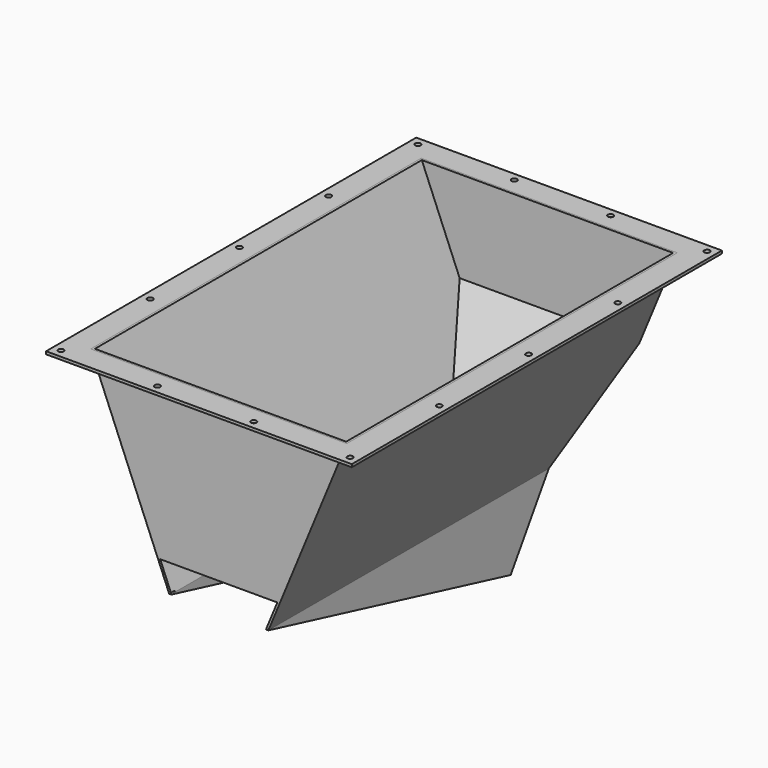
from build123d import *

# Parameters (mm, degrees)
F1_DEPTH  = 1500
F2_W      = 1110
F2_H      = 1680
F2_W_2    = 930
F2_H_2    = 1500
F3_DEPTH  = 10
F4_R      = 10
F5_DEPTH  = 10
F7_DEPTH  = 1110.001
F8_T      = -8
F10_DEPTH = 8
F11_W     = 344
F11_H     = 1124.6517558367
F12_DEPTH = 8


with BuildPart() as f1:
    # F0 (on Front) → F1 (new body)
    with BuildSketch(Plane.XZ):
        Polygon((465, 560), (-465, 560), (-180, -130), (-180, -400), (180, -400), (180, -130), align=None)
    extrude(amount=-F1_DEPTH)

    # F6 (on face) → F7 (cut, through all)
    with BuildSketch(Plane.YZ.offset(555)):
        Polygon((0, -400), (1100, -400), (0, -130), align=None)
        Polygon((1500, 225), (1100, -400), (1500, -400), align=None)
    extrude(amount=-F7_DEPTH, mode=Mode.SUBTRACT)

    # F8
    f8_openings = [f1.faces().sort_by_distance(p)[0] for p in [
        (0, 750, 560),
    ]]
    offset(amount=F8_T, openings=f8_openings, kind=Kind.INTERSECTION)

    # F9 (on Front) → F10 (cut)
    with BuildSketch(Plane.XZ):
        Polygon((212.6487880778, -30), (-212.6487880778, -30), (-171.3444402517, -130), (171.3444402517, -130), align=None)
    extrude(amount=-F10_DEPTH, mode=Mode.SUBTRACT)

    # F11 (on face) → F12 (cut)
    with BuildSketch(Plane(origin=(0, -30.0958765297, -122.6128303063), x_dir=(1, 0, 0), z_dir=(0, -0.2383786531, -0.9711722905))):
        with Locations((0, -593.3151028228)):
            Rectangle(F11_W, F11_H)
    extrude(amount=-F12_DEPTH, mode=Mode.SUBTRACT)


with BuildPart() as f3:
    # F2 (on face) → F3 (new body)
    with BuildSketch(Plane.XY.offset(560)):
        with Locations((0, 750)):
            Rectangle(F2_W, F2_H)
        with Locations((0, 750)):
            Rectangle(F2_W_2, F2_H_2, mode=Mode.SUBTRACT)
    extrude(amount=-F3_DEPTH)

    # F4 (on face) → F5 (cut)
    with BuildSketch(Plane.XY.offset(560)):
        with Locations((-525, 1560)):
            Circle(F4_R)
        with Locations((-175, 1560)):
            Circle(F4_R)
        with Locations((175, 1560)):
            Circle(F4_R)
        with Locations((525, 1560)):
            Circle(F4_R)
        with Locations((525, 1155)):
            Circle(F4_R)
        with Locations((525, 750)):
            Circle(F4_R)
        with Locations((525, 345)):
            Circle(F4_R)
        with Locations((525, -60)):
            Circle(F4_R)
        with Locations((-525, 1155)):
            Circle(F4_R)
        with Locations((-525, 750)):
            Circle(F4_R)
        with Locations((-525, 345)):
            Circle(F4_R)
        with Locations((-525, -60)):
            Circle(F4_R)
        with Locations((175, -60)):
            Circle(F4_R)
        with Locations((-175, -60)):
            Circle(F4_R)
    extrude(amount=-F5_DEPTH, mode=Mode.SUBTRACT)


solid = Compound([f1.part, f3.part])
